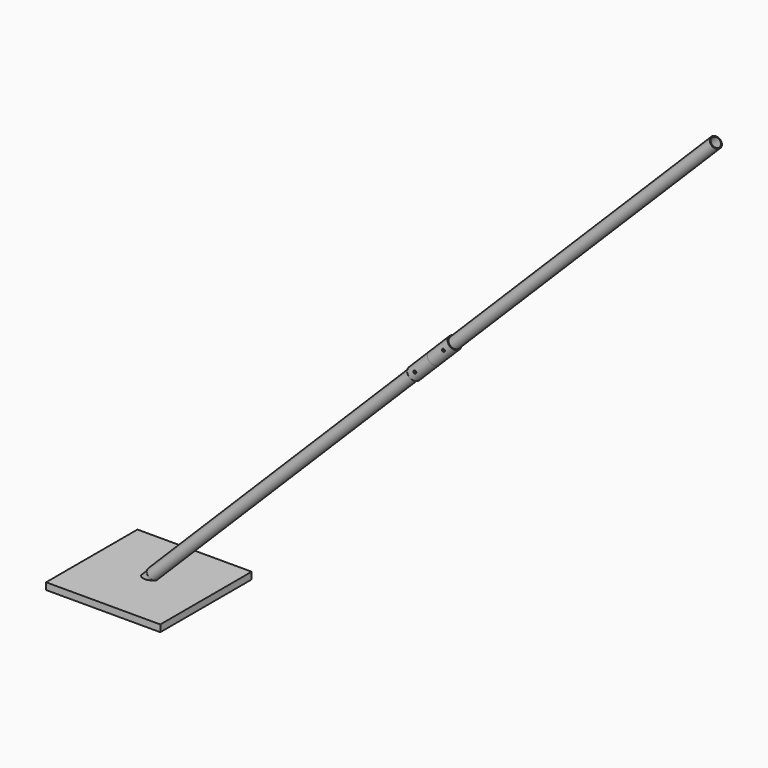
from build123d import *

# Parameters (mm, degrees)
F0_W           = 400
F0_H           = 400
F1_DEPTH       = 24
F10_R          = 5
F11_DEPTH      = 200.001
F11_DEPTH_BACK = 200.001


with BuildPart() as f1:
    # F0 (on Top) → F1 (new body)
    with BuildSketch(Plane.XY):
        Rectangle(F0_W, F0_H)
    extrude(amount=-F1_DEPTH)

    # F3 (on offset) → F4 (revolve)
    with BuildSketch(Plane.XZ):
        Polygon((343.6538956567, 363.4528855299), (341.5325753131, 365.5742058734), (-24.0416305603, 0), (-19.7989898732, 0), align=None)
    revolve(axis=Axis((176.7766952966, 0, 176.7766952966), (0.7071067812, 0, 0.7071067812)))


with BuildPart() as f6:
    # F5 (on offset) → F6 (revolve)
    with BuildSketch(Plane.XZ):
        Polygon((1973.8370490961, 1997.8786796564), (1971.7157287525, 2000), (0, 28.2842712475), (2.1213203436, 26.1629509039), align=None)
    revolve(axis=Axis((1000, 0, 1000), (0.7071067812, 0, 0.7071067812)))


with BuildPart() as f8:
    # F7 (on offset) → F8 (revolve)
    with BuildSketch(Plane.XZ):
        Polygon((985.8578643763, 1014.1421356237), (1056.5685424949, 1084.8528137424), (1054.4472221514, 1086.9741340859), (983.7365440327, 1016.2634559673), align=None)
    revolve(axis=Axis((1035.3553390593, 0, 1035.3553390593), (0.7071067812, 0, 0.7071067812)))

    # F9: F8 across face


with BuildPart() as f8_1:
    add(f8.part)
    add(f8.part.mirror(Plane(origin=(1000, 0, 1000), x_dir=(0, -1, 0), z_dir=(-0.7071067812, 0, -0.7071067812))))


with BuildPart() as f11_tool:
    # F10 (on offset) → F11 (new body, two sides)
    with BuildSketch(Plane.XZ) as f11_sk:
        with Locations((950, 950)):
            Circle(F10_R)
        with Locations((1050, 1050)):
            Circle(F10_R)
    extrude(amount=-F11_DEPTH)
    extrude(f11_sk.sketch, amount=F11_DEPTH_BACK)


with BuildPart() as f6_1:
    add(f6.part)

    # F11: cut by f11_tool
    add(f11_tool.part, mode=Mode.SUBTRACT)


with BuildPart() as f8_2:
    add(f8_1.part)

    # F11: cut by f11_tool
    add(f11_tool.part, mode=Mode.SUBTRACT)


solid = Compound([f1.part, f6_1.part, f8_2.part])
